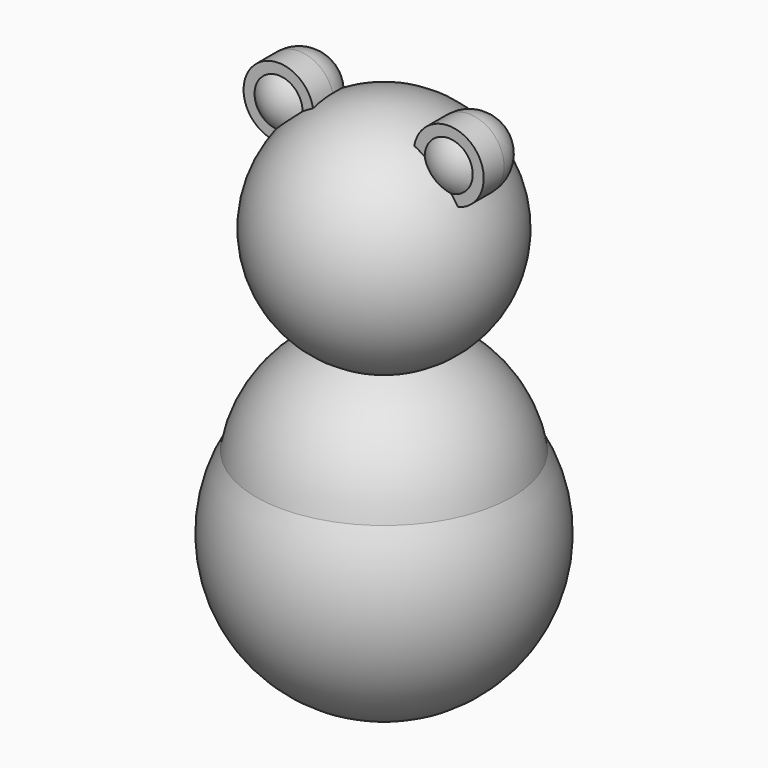
from build123d import *

# Parameters (mm, degrees)
F2_R     = 27.5
F3_DEPTH = 20


# Not quite as in the source:
# - a feature names something its author has since deleted; it is built from what else it names


with BuildPart() as f1:
    # F0 (on Front) → F1 (revolve)
    with BuildSketch(Plane.XZ):
        with BuildLine():
            Line((0, -90), (0, 90))
            ThreePointArc((0, 90), (-90, 0), (0, -90))
        make_face()
    revolve(axis=Axis((0, 0, 3.2690457241), (0, 0, -1)))

    # F2 (on Front) → F3 (join)
    with BuildSketch(Plane.XZ):
        with Locations((-66.8500438333, 73.4359920025)):
            Circle(F2_R)
        with Locations((66.8500438333, 73.4359920025)):
            Circle(F2_R)
    extrude(amount=F3_DEPTH)

    # F4 (on face) → F5 (revolve)
    with BuildSketch(Plane(origin=(0, 0, 0), x_dir=(-1, 0, 0), z_dir=(0, 1, 0))):
        with BuildLine():
            Line((66.8500438333, 100.9359920025), (66.8500438333, 45.9359920025))
            ThreePointArc((66.8500438333, 45.9359920025), (94.3500438333, 73.4359920025), (66.8500438333, 100.9359920025))
        make_face()
    revolve(axis=Axis((-66.8500438333, 0, 71.019994095), (0, 0, -1)))

    # F6 (on face) → F7 (revolve)
    with BuildSketch(Plane(origin=(0, 0, 0), x_dir=(-1, 0, 0), z_dir=(0, 1, 0))):
        with BuildLine():
            Line((-66.8500438333, 100.9359920025), (-66.8500438333, 45.9359920025))
            ThreePointArc((-66.8500438333, 45.9359920025), (-39.3500438333, 73.4359920025), (-66.8500438333, 100.9359920025))
        make_face()
    revolve(axis=Axis((66.8500438333, 0, 79.5244728215), (0, 0, -1)))

    # F8 (on Right) → F9 (revolve)
    with BuildSketch(Plane.YZ):
        with BuildLine():
            ThreePointArc((0, -326.6847895979), (100.2179567321, -268.9169130562), (100.4595458508, -153.2419025898))
            ThreePointArc((100.4595458508, -153.2419025898), (65.487785005, -92.9832219274), (0, -69.2033424707))
            Line((0, -69.2033424707), (0, -326.6847895979))
        make_face()
    revolve(axis=Axis((0, 0, -34.6016712354), (0, 0, -1)))


solid = f1.part
